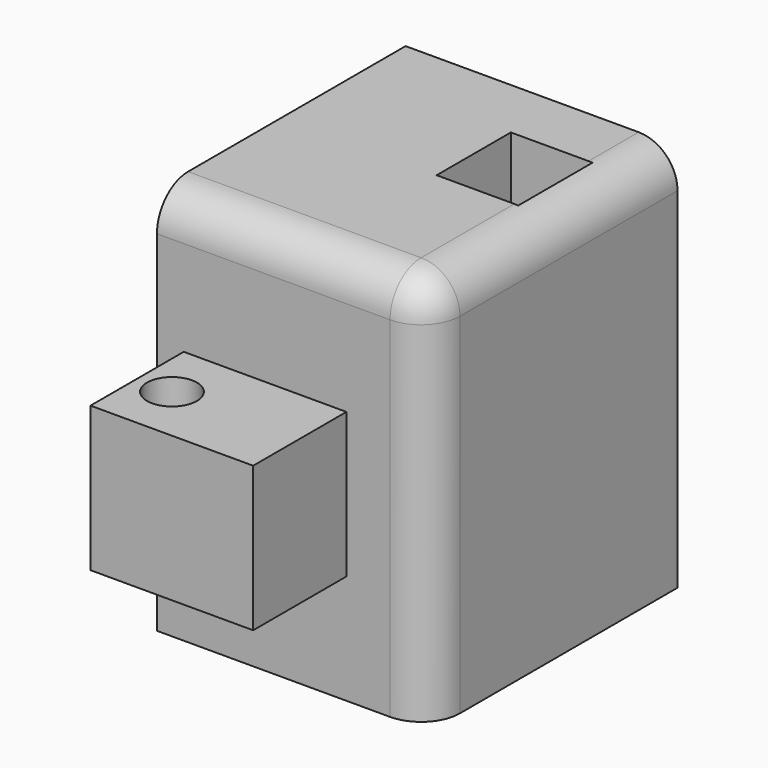
from build123d import *

# Parameters (mm, degrees)
F0_W         = 70
F0_H         = 80
F0_W_2       = 20.9936025798
F0_H_2       = 23.8757147082
F1_DEPTH     = 100
F2_W         = 41.873505339
F2_H         = 37.2992325574
F3_DEPTH     = 30
F4_R         = 6.4210037994
F5_DEPTH     = 50
F6_T1_DEPTH  = 85
F6_T3_DEPTH  = 95
F6_T5_DEPTH  = 115
F6_S9_W      = 10
F6_S9_H      = 10
F6_T10_DEPTH = 10


# Not quite as in the source:
# - a fillet or chamfer that OpenCascade refuses, or shapes differently, is made with other operations: its cross-section is extruded or revolved along the edge and cut away or added


with BuildPart() as f1:
    # F0 (on Top) → F1 (new body)
    with BuildSketch(Plane.XY):
        with Locations((-5.7970939631, 1.8514618278)):
            Rectangle(F0_W, F0_H)
        with Locations((9.6997073268, 13.7893191818)):
            Rectangle(F0_W_2, F0_H_2, mode=Mode.SUBTRACT)
    extrude(amount=F1_DEPTH)

    # F2 (on face) → F3 (join)
    with BuildSketch(Plane.XZ.offset(38.1485381722)):
        with Locations((-12.9710743204, 46.823351644)):
            Rectangle(F2_W, F2_H)
    extrude(amount=F3_DEPTH)

    # F4 (on face) → F5 (cut)
    with BuildSketch(Plane.XY.offset(65.4729679227)):
        with Locations((-24.8845424503, -53.2096363604)):
            Circle(F4_R)
    extrude(amount=-F5_DEPTH, mode=Mode.SUBTRACT)

    # F6: fillet of radius 10 on 3 edges, made by hand

    # F6_s2 → F6_t1 (cut)
    with BuildSketch(Plane.YZ.offset(-65.7970939631)):
        with BuildLine():
            ThreePointArc((-28.1485381722, 100), (-35.2196059841, 97.0710678119), (-38.1485381722, 90))
            Line((-38.1485381722, 90), (-38.1485381722, 100))
            Line((-38.1485381722, 100), (-28.1485381722, 100))
        make_face()
    extrude(amount=F6_T1_DEPTH, mode=Mode.SUBTRACT)

    # F6_s4 → F6_t3 (cut)
    with BuildSketch(Plane.XZ.offset(-66.8514618278)):
        with BuildLine():
            ThreePointArc((29.2029060369, 90), (26.2739738488, 97.0710678119), (19.2029060369, 100))
            Line((19.2029060369, 100), (29.2029060369, 100))
            Line((29.2029060369, 100), (29.2029060369, 90))
        make_face()
    extrude(amount=F6_T3_DEPTH, mode=Mode.SUBTRACT)

    # F6_s6 → F6_t5 (cut)
    with BuildSketch(Plane.XY.offset(-25)):
        with BuildLine():
            ThreePointArc((29.2029060369, -28.1485381722), (26.2739738488, -35.2196059841), (19.2029060369, -38.1485381722))
            Line((19.2029060369, -38.1485381722), (29.2029060369, -38.1485381722))
            Line((29.2029060369, -38.1485381722), (29.2029060369, -28.1485381722))
        make_face()
    extrude(amount=F6_T5_DEPTH, mode=Mode.SUBTRACT)


with BuildPart() as f6_tool8:
    # F6_s9 → F6_t10 (new body)
    with BuildSketch(Plane.YZ.offset(19.2029060369)):
        with Locations((-33.1485381722, 95)):
            Rectangle(F6_S9_W, F6_S9_H)
    extrude(amount=F6_T10_DEPTH)

    # F6_s11 → F6_t12 (revolve, cut)
    with BuildSketch(Plane(origin=(19.2029060369, -28.1485381722, 90), x_dir=(0, 0.7071067812, -0.7071067812), z_dir=(0, -0.7071067812, -0.7071067812))):
        with BuildLine():
            ThreePointArc((0, -10), (10, 0), (0, 10))
            Line((0, 10), (0, -10))
        make_face()
    revolve(axis=Axis((19.2029060369, -28.1485381722, 90), (1, 0, 0)), mode=Mode.SUBTRACT)


with BuildPart() as f1_1:
    add(f1.part)

    # F6_t7: cut F6_tool8
    add(f6_tool8.part, mode=Mode.SUBTRACT)


solid = f1_1.part
